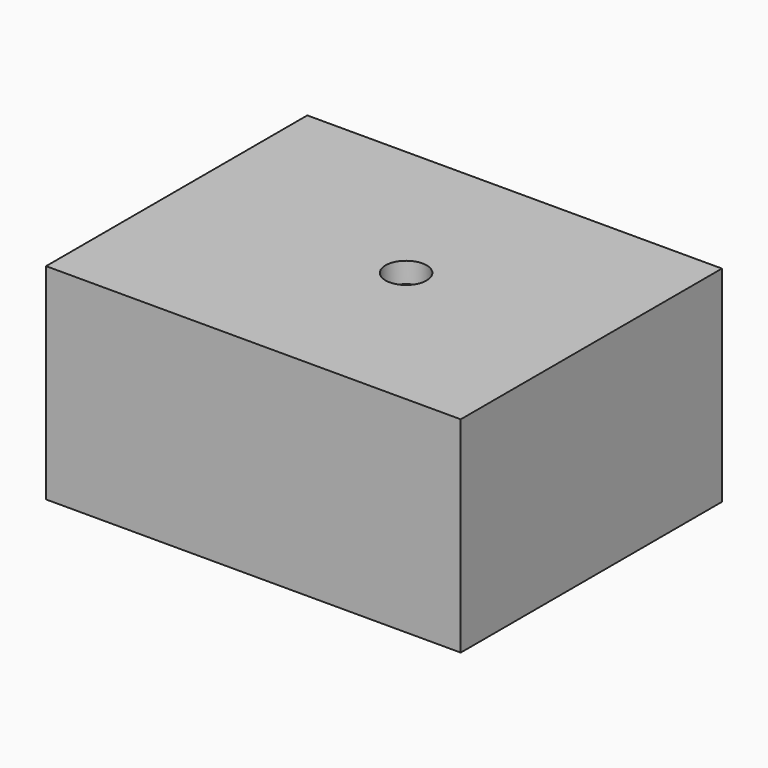
from build123d import *

# Parameters (mm, degrees)
F0_W           = 51.2767769396
F0_H           = 40.3746776283
F1_DEPTH       = 25.4
F2_W           = 14.1758769751
F2_H           = 15.7698839903
F3_DEPTH       = 12.7
F4_T           = -2.54
F5_SIZE        = 2.53999
F7_D           = 2.54
F7_CBORE_D     = 5.08
F7_CBORE_DEPTH = 2.54


# Not quite as in the source:
# - a fillet or chamfer is up to 0.001 mm smaller than in the source, because OpenCascade refuses the exact size


with BuildPart() as f1:
    # F0 (on Top) → F1 (new body)
    with BuildSketch(Plane.XY):
        with Locations((25.6383884698, 20.1873388141)):
            Rectangle(F0_W, F0_H)
    extrude(amount=F1_DEPTH)

    # F2 (on face) → F3 (join)
    with BuildSketch(Plane.XY.offset(25.4)):
        with Locations((19.3085148931, 20.5943360925)):
            Rectangle(F2_W, F2_H)
    extrude(amount=-F3_DEPTH)

    # F4
    f4_openings = [f1.faces().sort_by_distance(p)[0] for p in [
        (25.638388, 20.187339, 0),
    ]]
    offset(amount=F4_T, openings=f4_openings)

    # F5 (size 2.54 in the source; OpenCascade refuses exactly that, so slightly less here)
    f5_edges = [f1.edges().sort_by_distance(p)[0] for p in [
        (2.54, 20.187339, 0),
        (25.638388, 37.834678, 0),
        (48.736777, 20.187339, 0),
        (25.638388, 2.54, 0),
    ]]
    chamfer(f5_edges, length=F5_SIZE)

    # F7 (through all)
    with Locations(Plane(origin=(0, 0, 22.86), x_dir=(1, 0, 0), z_dir=(0, 0, -1))):
        with Locations((28.0292164534, -20.6155125052)):
            CounterBoreHole(F7_D / 2, F7_CBORE_D / 2, F7_CBORE_DEPTH)


solid = f1.part
